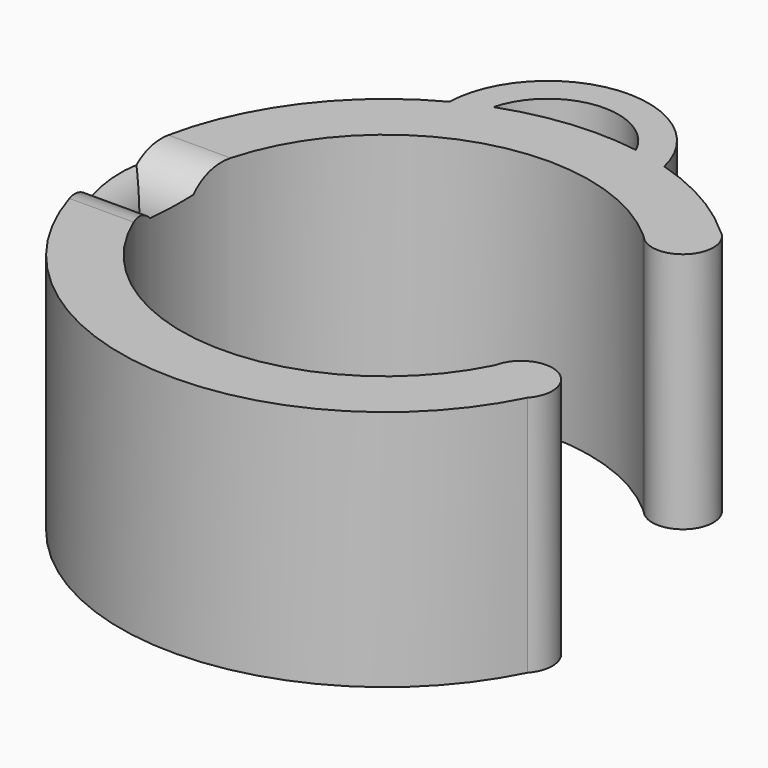
from build123d import *

# Parameters (mm, degrees)
F0_W         = 3.7644430995
F0_H         = 3.6893493962
F1_DEPTH     = 25.4
F3_DEPTH     = 25.4
F4_T1_DEPTH  = 3.6893493962
F5_T1_DEPTH  = 3.6893493962
F6_T4_DEPTH  = 31.7513819576
F6_S5_R      = 5.0800000001
F6_T6_DEPTH  = 18
F6_S7_R      = 5.0799999999
F6_T8_DEPTH  = 18
F6_T12_DEPTH = 31.8046354707
F6_S13_R     = 5.0800000001
F6_T14_DEPTH = 18
F6_S15_R     = 5.0799999999
F6_T16_DEPTH = 18
F7_T1_DEPTH  = 3.6893493962
F7_T3_DEPTH  = 3.7644430995
F7_T9_DEPTH  = 16.3893493962
F7_S11_R     = 27.7843331243
F7_T12_DEPTH = 10
F7_T15_DEPTH = 16.4644430995
F7_S17_R     = 27.7843331243
F7_T18_DEPTH = 10
F7_T24_DEPTH = 16.4644430995
F7_S26_R     = 27.7843331243
F7_T27_DEPTH = 10
F7_T30_DEPTH = 16.3893493962
F7_S32_R     = 27.7843331243
F7_T33_DEPTH = 10
F7_T39_DEPTH = 16.3893493962
F7_S41_R     = 21.4343331243
F7_T42_DEPTH = 10
F7_T45_DEPTH = 16.4644430995
F7_S47_R     = 21.4343331243
F7_T48_DEPTH = 10
F7_T54_DEPTH = 16.3893493962
F7_S56_R     = 21.4343331243
F7_T57_DEPTH = 10
F7_T60_DEPTH = 16.4644430995
F7_S62_R     = 21.4343331243
F7_T63_DEPTH = 10


# Not quite as in the source:
# - a fillet or chamfer that OpenCascade refuses, or shapes differently, is made with other operations: its cross-section is extruded or revolved along the edge and cut away or added


with BuildPart() as f1:
    # F0 (on Top) → F1 (new body)
    with BuildSketch(Plane.XY):
        with BuildLine():
            ThreePointArc((21.5192791075, -12.0412250981), (-18.6952618922, -6.6001770911), (16.4842832794, 13.628859286))
            ThreePointArc((16.4842832794, 13.628859286), (16.7004899528, 13.4298852219), (16.9072606144, 13.2211224445))
            ThreePointArc((16.9072606144, 13.2211224445), (21.6662962935, 13.3359323022), (21.0575650897, 18.0572719658))
            ThreePointArc((21.0575650897, 18.0572719658), (-24.9747625183, -7.5703236346), (27.2017178865, -14.8753721518))
            ThreePointArc((27.2017178865, -14.8753721518), (26.2135164235, -9.7430147231), (21.5192791075, -12.0412250981))
        make_face()
        with Locations((-21.9849217683, -3.8102302933)):
            Rectangle(F0_W, F0_H, mode=Mode.SUBTRACT)
    extrude(amount=F1_DEPTH)

    # F2 (on Top) → F3 (join)
    with BuildSketch(Plane.XY):
        with BuildLine():
            ThreePointArc((-7.1930247185, 23.6237348024), (-0.7260554424, 29.1452143248), (6.6808082429, 24.968277878))
            ThreePointArc((6.6808082429, 24.968277878), (8.51162891, 24.6152301343), (10.3146480708, 24.140183894))
            ThreePointArc((10.3146480708, 24.140183894), (-1.0323167037, 32.3054087872), (-10.6002305361, 22.1132778988))
            ThreePointArc((-10.6002305361, 22.1132778988), (-8.9219828274, 22.9257012198), (-7.1930247185, 23.6237348025))
        make_face()
    extrude(amount=F3_DEPTH)

    # F4: fillet of radius 5.08 on 1 edges, made by hand

    # F4_s2 → F4_t1 (cut)
    with BuildSketch(Plane.XZ.offset(1.9655555952)):
        with BuildLine():
            ThreePointArc((-15.0227002186, 25.4), (-18.614802667, 23.9121024484), (-20.1027002186, 20.32))
            Line((-20.1027002186, 20.32), (-20.1027002186, 25.4))
            Line((-20.1027002186, 25.4), (-15.0227002186, 25.4))
        make_face()
    extrude(amount=F4_T1_DEPTH, mode=Mode.SUBTRACT)

    # F5: fillet of radius 5.08 on 1 edges, made by hand

    # F5_s2 → F5_t1 (cut)
    with BuildSketch(Plane.XZ.offset(1.9655555952)):
        with BuildLine():
            ThreePointArc((-28.9471433181, 25.4), (-25.3550408696, 23.9121024484), (-23.8671433181, 20.32))
            Line((-23.8671433181, 20.32), (-23.8671433181, 25.4))
            Line((-23.8671433181, 25.4), (-28.9471433181, 25.4))
        make_face()
    extrude(amount=F5_T1_DEPTH, mode=Mode.SUBTRACT)

    # F6: fillet of radius 5.08 on 2 edges, made by hand


with BuildPart() as f6_tool2:
    # F6_s3 → F6_t4 (new body)
    with BuildSketch(Plane.YZ.offset(-6.3899983285)):
        with BuildLine():
            ThreePointArc((-1.9655555952, 20.32), (-0.4776580437, 23.9121024484), (3.1144444048, 25.4))
            Line((3.1144444048, 25.4), (-1.9655555952, 25.4))
            Line((-1.9655555952, 25.4), (-1.9655555952, 20.32))
        make_face()
    extrude(amount=-F6_T4_DEPTH)

    # F6_s5 → F6_t6 (cut, symmetric)
    with BuildSketch(Plane.XZ.offset(-0.6)):
        with Locations((-15.0227002185, 20.3199999999)):
            Circle(F6_S5_R)
    extrude(amount=F6_T6_DEPTH, both=True, mode=Mode.SUBTRACT)

    # F6_s7 → F6_t8 (cut, symmetric)
    with BuildSketch(Plane.XZ.offset(-0.6)):
        with Locations((-28.947143318, 20.3200000001)):
            Circle(F6_S7_R)
    extrude(amount=F6_T8_DEPTH, both=True, mode=Mode.SUBTRACT)


with BuildPart() as f1_1:
    add(f1.part)

    # F6_t1: cut F6_tool2
    add(f6_tool2.part, mode=Mode.SUBTRACT)


with BuildPart() as f6_tool10:
    # F6_s11 → F6_t12 (new body)
    with BuildSketch(Plane.YZ.offset(-6.1587934503)):
        with BuildLine():
            ThreePointArc((-10.7349049914, 25.4), (-7.142802543, 23.9121024484), (-5.6549049914, 20.32))
            Line((-5.6549049914, 20.32), (-5.6549049914, 25.4))
            Line((-5.6549049914, 25.4), (-10.7349049914, 25.4))
        make_face()
    extrude(amount=-F6_T12_DEPTH)

    # F6_s13 → F6_t14 (cut, symmetric)
    with BuildSketch(Plane.XZ.offset(8.2)):
        with Locations((-15.0227002185, 20.3199999999)):
            Circle(F6_S13_R)
    extrude(amount=F6_T14_DEPTH, both=True, mode=Mode.SUBTRACT)

    # F6_s15 → F6_t16 (cut, symmetric)
    with BuildSketch(Plane.XZ.offset(8.2)):
        with Locations((-28.947143318, 20.3200000001)):
            Circle(F6_S15_R)
    extrude(amount=F6_T16_DEPTH, both=True, mode=Mode.SUBTRACT)


with BuildPart() as f1_2:
    add(f1_1.part)

    # F6_t9: cut F6_tool10
    add(f6_tool10.part, mode=Mode.SUBTRACT)

    # F7: fillet of radius 5.08 on 4 edges, made by hand

    # F7_s2 → F7_t1 (cut)
    with BuildSketch(Plane.XZ.offset(1.9655555952)):
        with BuildLine():
            ThreePointArc((-23.8671433181, 5.08), (-25.3550408696, 1.4878975516), (-28.9471433181, 0))
            Line((-28.9471433181, 0), (-23.8671433181, 0))
            Line((-23.8671433181, 0), (-23.8671433181, 5.08))
        make_face()
        with BuildLine():
            ThreePointArc((-20.1027002186, 5.08), (-18.614802667, 1.4878975516), (-15.0227002186, 0))
            Line((-15.0227002186, 0), (-20.1027002186, 0))
            Line((-20.1027002186, 0), (-20.1027002186, 5.08))
        make_face()
    extrude(amount=F7_T1_DEPTH, mode=Mode.SUBTRACT)

    # F7_s4 → F7_t3 (cut)
    with BuildSketch(Plane.YZ.offset(-23.8671433181)):
        with BuildLine():
            ThreePointArc((-5.6549049914, 5.08), (-7.142802543, 1.4878975516), (-10.7349049914, 0))
            Line((-10.7349049914, 0), (-5.6549049914, 0))
            Line((-5.6549049914, 0), (-5.6549049914, 5.08))
        make_face()
        with BuildLine():
            ThreePointArc((-1.9655555952, 5.08), (-0.4776580437, 1.4878975516), (3.1144444048, 0))
            Line((3.1144444048, 0), (-1.9655555952, 0))
            Line((-1.9655555952, 0), (-1.9655555952, 5.08))
        make_face()
    extrude(amount=F7_T3_DEPTH, mode=Mode.SUBTRACT)


with BuildPart() as f7_tool7:
    # F7_s8 → F7_t9 (new body)
    with BuildSketch(Plane.XZ.offset(18.3549049914)):
        with BuildLine():
            ThreePointArc((-23.8671433181, 5.08), (-25.3550408696, 1.4878975516), (-28.9471433181, 0))
            Line((-28.9471433181, 0), (-23.8671433181, 0))
            Line((-23.8671433181, 0), (-23.8671433181, 5.08))
        make_face()
    extrude(amount=-F7_T9_DEPTH)

    split(bisect_by=Plane.XZ.offset(5.6549049914), keep=Keep.TOP)

    # F7_s11 → F7_t12 (intersect, symmetric)
    with BuildSketch(Plane.XY.offset(2.5)):
        with Locations((2.3382892257, -2.4746027243)):
            Circle(F7_S11_R)
    extrude(amount=F7_T12_DEPTH, both=True, mode=Mode.INTERSECT)


with BuildPart() as f7_tool13:
    # F7_s14 → F7_t15 (new body)
    with BuildSketch(Plane.YZ.offset(-20.1027002186)):
        with BuildLine():
            ThreePointArc((-5.6549049914, 5.08), (-7.142802543, 1.4878975516), (-10.7349049914, 0))
            Line((-10.7349049914, 0), (-5.6549049914, 0))
            Line((-5.6549049914, 0), (-5.6549049914, 5.08))
        make_face()
    extrude(amount=-F7_T15_DEPTH)

    split(bisect_by=Plane.YZ.offset(-23.8671433181), keep=Keep.BOTTOM)

    # F7_s17 → F7_t18 (intersect, symmetric)
    with BuildSketch(Plane.XY.offset(2.5)):
        with Locations((2.3382892257, -2.4746027243)):
            Circle(F7_S17_R)
    extrude(amount=F7_T18_DEPTH, both=True, mode=Mode.INTERSECT)


with BuildPart() as f7_tool7_1:
    add(f7_tool7.part)

    # F7_t19: intersect F7_tool13
    add(f7_tool13.part, mode=Mode.INTERSECT)


with BuildPart() as f1_3:
    add(f1_2.part)

    # F7_t5: cut F7_tool7
    add(f7_tool7_1.part, mode=Mode.SUBTRACT)


with BuildPart() as f7_tool22:
    # F7_s23 → F7_t24 (new body)
    with BuildSketch(Plane.YZ.offset(-36.5671433181)):
        with BuildLine():
            ThreePointArc((-1.9655555952, 5.08), (-0.4776580437, 1.4878975516), (3.1144444048, 0))
            Line((3.1144444048, 0), (-1.9655555952, 0))
            Line((-1.9655555952, 0), (-1.9655555952, 5.08))
        make_face()
    extrude(amount=F7_T24_DEPTH)

    split(bisect_by=Plane.YZ.offset(-23.8671433181), keep=Keep.BOTTOM)

    # F7_s26 → F7_t27 (intersect, symmetric)
    with BuildSketch(Plane.XY.offset(2.5)):
        with Locations((2.3382892257, -2.4746027243)):
            Circle(F7_S26_R)
    extrude(amount=F7_T27_DEPTH, both=True, mode=Mode.INTERSECT)


with BuildPart() as f7_tool28:
    # F7_s29 → F7_t30 (new body)
    with BuildSketch(Plane.XZ.offset(5.6549049914)):
        with BuildLine():
            ThreePointArc((-23.8671433181, 5.08), (-25.3550408696, 1.4878975516), (-28.9471433181, 0))
            Line((-28.9471433181, 0), (-23.8671433181, 0))
            Line((-23.8671433181, 0), (-23.8671433181, 5.08))
        make_face()
    extrude(amount=-F7_T30_DEPTH)

    split(bisect_by=Plane.XZ.offset(1.9655555952), keep=Keep.BOTTOM)

    # F7_s32 → F7_t33 (intersect, symmetric)
    with BuildSketch(Plane.XY.offset(2.5)):
        with Locations((2.3382892257, -2.4746027243)):
            Circle(F7_S32_R)
    extrude(amount=F7_T33_DEPTH, both=True, mode=Mode.INTERSECT)


with BuildPart() as f7_tool22_1:
    add(f7_tool22.part)

    # F7_t34: intersect F7_tool28
    add(f7_tool28.part, mode=Mode.INTERSECT)


with BuildPart() as f1_4:
    add(f1_3.part)

    # F7_t20: cut F7_tool22
    add(f7_tool22_1.part, mode=Mode.SUBTRACT)


with BuildPart() as f7_tool37:
    # F7_s38 → F7_t39 (new body)
    with BuildSketch(Plane.XZ.offset(-10.7344444048)):
        with BuildLine():
            ThreePointArc((-20.1027002186, 5.08), (-18.614802667, 1.4878975516), (-15.0227002186, 0))
            Line((-15.0227002186, 0), (-20.1027002186, 0))
            Line((-20.1027002186, 0), (-20.1027002186, 5.08))
        make_face()
    extrude(amount=F7_T39_DEPTH)

    split(bisect_by=Plane.XZ.offset(1.9655555952), keep=Keep.BOTTOM)

    # F7_s41 → F7_t42 (cut, symmetric)
    with BuildSketch(Plane.XY.offset(2.5)):
        with Locations((2.3382892257, -2.4746027243)):
            Circle(F7_S41_R)
    extrude(amount=F7_T42_DEPTH, both=True, mode=Mode.SUBTRACT)


with BuildPart() as f7_tool43:
    # F7_s44 → F7_t45 (new body)
    with BuildSketch(Plane.YZ.offset(-23.8671433181)):
        with BuildLine():
            ThreePointArc((-1.9655555952, 5.08), (-0.4776580437, 1.4878975516), (3.1144444048, 0))
            Line((3.1144444048, 0), (-1.9655555952, 0))
            Line((-1.9655555952, 0), (-1.9655555952, 5.08))
        make_face()
    extrude(amount=F7_T45_DEPTH)

    split(bisect_by=Plane.YZ.offset(-20.1027002186), keep=Keep.TOP)

    # F7_s47 → F7_t48 (cut, symmetric)
    with BuildSketch(Plane.XY.offset(2.5)):
        with Locations((2.3382892257, -2.4746027243)):
            Circle(F7_S47_R)
    extrude(amount=F7_T48_DEPTH, both=True, mode=Mode.SUBTRACT)


with BuildPart() as f7_tool37_1:
    add(f7_tool37.part)

    # F7_t49: intersect F7_tool43
    add(f7_tool43.part, mode=Mode.INTERSECT)


with BuildPart() as f1_5:
    add(f1_4.part)

    # F7_t35: cut F7_tool37
    add(f7_tool37_1.part, mode=Mode.SUBTRACT)


with BuildPart() as f7_tool52:
    # F7_s53 → F7_t54 (new body)
    with BuildSketch(Plane.XZ.offset(1.9655555952)):
        with BuildLine():
            ThreePointArc((-20.1027002186, 5.08), (-18.614802667, 1.4878975516), (-15.0227002186, 0))
            Line((-15.0227002186, 0), (-20.1027002186, 0))
            Line((-20.1027002186, 0), (-20.1027002186, 5.08))
        make_face()
    extrude(amount=F7_T54_DEPTH)

    split(bisect_by=Plane.XZ.offset(5.6549049914), keep=Keep.TOP)

    # F7_s56 → F7_t57 (cut, symmetric)
    with BuildSketch(Plane.XY.offset(2.5)):
        with Locations((2.3382892257, -2.4746027243)):
            Circle(F7_S56_R)
    extrude(amount=F7_T57_DEPTH, both=True, mode=Mode.SUBTRACT)


with BuildPart() as f7_tool58:
    # F7_s59 → F7_t60 (new body)
    with BuildSketch(Plane.YZ.offset(-7.4027002186)):
        with BuildLine():
            ThreePointArc((-5.6549049914, 5.08), (-7.142802543, 1.4878975516), (-10.7349049914, 0))
            Line((-10.7349049914, 0), (-5.6549049914, 0))
            Line((-5.6549049914, 0), (-5.6549049914, 5.08))
        make_face()
    extrude(amount=-F7_T60_DEPTH)

    split(bisect_by=Plane.YZ.offset(-20.1027002186), keep=Keep.TOP)

    # F7_s62 → F7_t63 (cut, symmetric)
    with BuildSketch(Plane.XY.offset(2.5)):
        with Locations((2.3382892257, -2.4746027243)):
            Circle(F7_S62_R)
    extrude(amount=F7_T63_DEPTH, both=True, mode=Mode.SUBTRACT)


with BuildPart() as f7_tool52_1:
    add(f7_tool52.part)

    # F7_t64: intersect F7_tool58
    add(f7_tool58.part, mode=Mode.INTERSECT)


with BuildPart() as f1_6:
    add(f1_5.part)

    # F7_t50: cut F7_tool52
    add(f7_tool52_1.part, mode=Mode.SUBTRACT)


solid = f1_6.part
